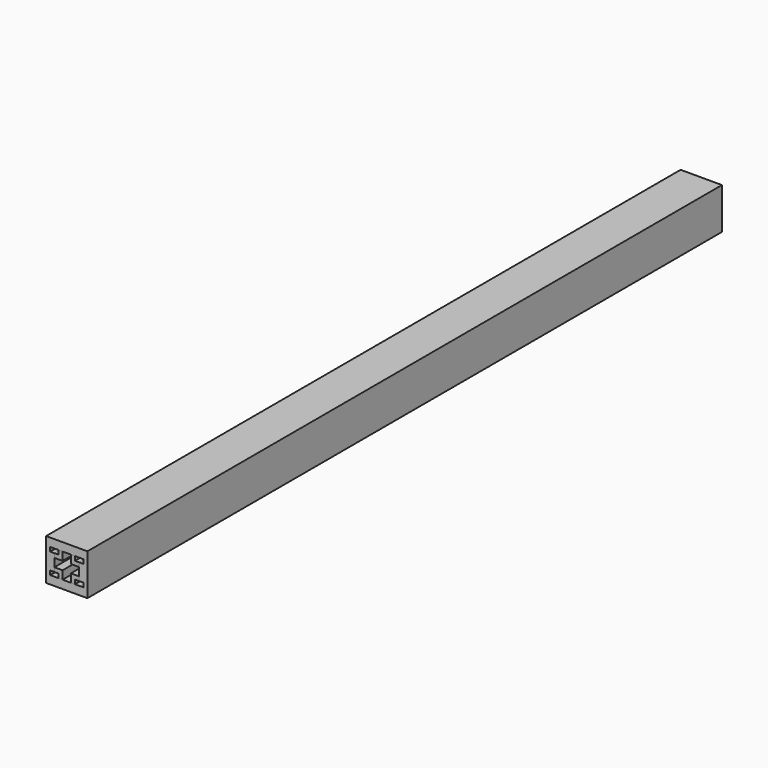
from build123d import *

# Parameters (mm, degrees)
F0_W      = 6.35
F0_H      = 609.6
F1_DEPTH  = 6.35
F2_DEPTH  = 12.7
F3_DEPTH  = 6.35
F4_W      = 31.75
F4_H      = 31.75
F4_W_2    = 19.05
F4_H_2    = 19.05
F5_DEPTH  = 609.6
F6_W      = 3.175
F6_H      = 3.175
F7_DEPTH  = 603.25
F8_W      = 3.175
F8_H      = 19.05
F9_DEPTH  = 12.7
F10_DEPTH = 6.35
F11_DEPTH = 12.7
F12_DEPTH = 6.35


with BuildPart() as f1:
    # F0 (on Top) → F1 (new body)
    with BuildSketch(Plane.XY):
        with Locations((-6.35, 304.8)):
            Rectangle(F0_W, F0_H)
    extrude(amount=F1_DEPTH)


with BuildPart() as f1b:
    # F0 (on Top) → F1, piece 2 (new body)
    with BuildSketch(Plane.XY):
        with Locations((6.35, 304.8)):
            Rectangle(F0_W, F0_H)
    extrude(amount=F1_DEPTH)


with BuildPart() as f2:
    # F0 (on Top) → F2 (new body)
    with BuildSketch(Plane.XY):
        with Locations((6.35, 304.8)):
            Rectangle(F0_W, F0_H)
    extrude(amount=-F2_DEPTH)


with BuildPart() as f2b:
    # F0 (on Top) → F2, piece 2 (new body)
    with BuildSketch(Plane.XY):
        with Locations((-6.35, 304.8)):
            Rectangle(F0_W, F0_H)
    extrude(amount=-F2_DEPTH)


with BuildPart() as f3_tool:
    # F0 (on Top) → F3 (new body)
    with BuildSketch(Plane.XY):
        with Locations((6.35, 304.8)):
            Rectangle(F0_W, F0_H)
        with Locations((-6.35, 304.8)):
            Rectangle(F0_W, F0_H)
    extrude(amount=-F3_DEPTH)


with BuildPart() as f2_1:
    add(f2.part)

    # F3: cut by f3_tool
    add(f3_tool.part, mode=Mode.SUBTRACT)


with BuildPart() as f2b_1:
    add(f2b.part)

    # F3: cut by f3_tool
    add(f3_tool.part, mode=Mode.SUBTRACT)


with BuildPart() as f5:
    # F4 (on Front) → F5 (new body)
    with BuildSketch(Plane.XZ):
        with Locations((0, -3.175)):
            Rectangle(F4_W, F4_H)
        with Locations((0, -3.175)):
            Rectangle(F4_W_2, F4_H_2, mode=Mode.SUBTRACT)
    extrude(amount=-F5_DEPTH)


with BuildPart() as f7_tool:
    # F6 (on face) → F7 (new body)
    with BuildSketch(Plane.XZ):
        with Locations((-11.1125, 4.7625)):
            Rectangle(F6_W, F6_H)
        with Locations((-7.9375, 4.7625)):
            Rectangle(F6_W, F6_H)
        with Locations((7.9375, 4.7625)):
            Rectangle(F6_W, F6_H)
        with Locations((11.1125, 4.7625)):
            Rectangle(F6_W, F6_H)
        with Locations((-11.1125, -11.1125)):
            Rectangle(F6_W, F6_H)
        with Locations((-7.9375, -11.1125)):
            Rectangle(F6_W, F6_H)
        with Locations((7.9375, -11.1125)):
            Rectangle(F6_W, F6_H)
        with Locations((11.1125, -11.1125)):
            Rectangle(F6_W, F6_H)
    extrude(amount=-F7_DEPTH)


with BuildPart() as f1_1:
    add(f1.part)

    # F7: cut by f7_tool
    add(f7_tool.part, mode=Mode.SUBTRACT)


with BuildPart() as f1b_1:
    add(f1b.part)

    # F7: cut by f7_tool
    add(f7_tool.part, mode=Mode.SUBTRACT)


with BuildPart() as f2_2:
    add(f2_1.part)

    # F7: cut by f7_tool
    add(f7_tool.part, mode=Mode.SUBTRACT)


with BuildPart() as f2b_2:
    add(f2b_1.part)

    # F7: cut by f7_tool
    add(f7_tool.part, mode=Mode.SUBTRACT)


with BuildPart() as f5_1:
    add(f5.part)

    # F7: cut by f7_tool
    add(f7_tool.part, mode=Mode.SUBTRACT)

    # F8 (on face) → F9 (cut)
    with BuildSketch(Plane(origin=(0, 609.6, 0), x_dir=(-1, 0, 0), z_dir=(0, 1, 0))):
        with Locations((-12.3825, -3.175)):
            Rectangle(F8_W, F8_H)
        with Locations((12.3825, -3.175)):
            Rectangle(F8_W, F8_H)
    extrude(amount=-F9_DEPTH, mode=Mode.SUBTRACT)

    # F8 (on face) → F10 (join)
    with BuildSketch(Plane(origin=(0, 609.6, 0), x_dir=(-1, 0, 0), z_dir=(0, 1, 0))):
        with Locations((-12.3825, -3.175)):
            Rectangle(F8_W, F8_H)
        with Locations((12.3825, -3.175)):
            Rectangle(F8_W, F8_H)
    extrude(amount=-F10_DEPTH)

    # F8 (on face) → F11 (cut)
    with BuildSketch(Plane(origin=(0, 609.6, 0), x_dir=(-1, 0, 0), z_dir=(0, 1, 0))):
        with Locations((12.3825, -3.175)):
            Rectangle(F8_W, F8_H)
    extrude(amount=-F11_DEPTH, mode=Mode.SUBTRACT)

    # F8 (on face) → F12 (join)
    with BuildSketch(Plane(origin=(0, 609.6, 0), x_dir=(-1, 0, 0), z_dir=(0, 1, 0))):
        with Locations((12.3825, -3.175)):
            Rectangle(F8_W, F8_H)
    extrude(amount=-F12_DEPTH)


solid = Compound([f1_1.part, f1b_1.part, f2_2.part, f2b_2.part, f5_1.part])
